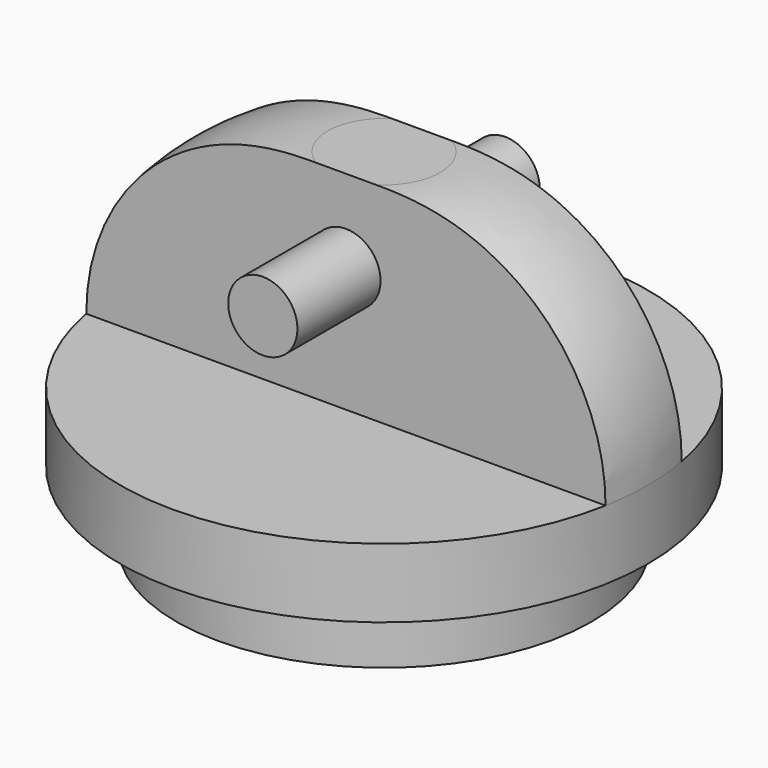
from build123d import *

# Parameters (mm, degrees)
F0_R        = 30
F1_DEPTH    = 10
F2_R        = 38.1255
F2_R_2      = 30
F3_DEPTH    = 10
F5_DEPTH    = 10
F7_DEPTH    = 20
F8_T2_ANGLE = 246.2138015041
F8_T4_ANGLE = 246.2138015041
F10_R       = 5
F11_DEPTH   = 15
F9_R        = 5
F12_DEPTH   = 15


# Not quite as in the source:
# - a fillet or chamfer that OpenCascade refuses, or shapes differently, is made with other operations: its cross-section is extruded or revolved along the edge and cut away or added


with BuildPart() as f1:
    # F0 (on Top) → F1 (new body)
    with BuildSketch(Plane.XY):
        Circle(F0_R)
    extrude(amount=F1_DEPTH)

    # F2 (on face) → F3 (join)
    with BuildSketch(Plane.XY.offset(10)):
        Circle(F2_R)
        Circle(F2_R_2, mode=Mode.SUBTRACT)
        Circle(F2_R_2)
    extrude(amount=F3_DEPTH)

    # F4 (on face) → F5 (join)
    with BuildSketch(Plane.XY.offset(20)):
        with BuildLine():
            Line((37.5, 6.8777721865), (-37.5, 6.8777721865))
            ThreePointArc((-37.5, 6.8777721865), (-38.1255, 0), (-37.5, -6.8777721865))
            Line((-37.5, -6.8777721865), (37.5, -6.8777721865))
            ThreePointArc((37.5, -6.8777721865), (37.9688029851, -3.4530783549), (38.1255, 0))
            ThreePointArc((38.1255, 0), (37.9688029851, 3.4530783549), (37.5, 6.8777721865))
        make_face()
    extrude(amount=F5_DEPTH)

    # F6 (on face) → F7 (join)
    with BuildSketch(Plane.XY.offset(30)):
        with BuildLine():
            Line((37.5, 6.8777721865), (-37.5, 6.8777721865))
            ThreePointArc((-37.5, 6.8777721865), (-38.1255, 0), (-37.5, -6.8777721865))
            Line((-37.5, -6.8777721865), (37.5, -6.8777721865))
            ThreePointArc((37.5, -6.8777721865), (38.1255, 0), (37.5, 6.8777721865))
        make_face()
    extrude(amount=F7_DEPTH)

    # F8: fillet of radius 30 on 2 edges, made by hand

    # F8_s1 → F8_t2 (revolve, cut)
    with BuildSketch(Plane(origin=(0, 0, 0), x_dir=(0, 0, 1), z_dir=(-0.8376529376, 0.5462028526, 0))):
        with BuildLine():
            ThreePointArc((20, -38.1255), (41.2132034356, -29.3387034356), (50, -8.1255))
            Line((50, -8.1255), (50, -38.1255))
            Line((50, -38.1255), (20, -38.1255))
        make_face()
    revolve(axis=Axis((0, 0, 50), (0, 0, 1)), revolution_arc=F8_T2_ANGLE, mode=Mode.SUBTRACT)

    # F8_s3 → F8_t4 (revolve, cut)
    with BuildSketch(Plane(origin=(0, 0, 0), x_dir=(0, 0, 1), z_dir=(0.8376529376, -0.5462028526, 0))):
        with BuildLine():
            ThreePointArc((20, -38.1255), (41.2132034356, -29.3387034356), (50, -8.1255))
            Line((50, -8.1255), (50, -38.1255))
            Line((50, -38.1255), (20, -38.1255))
        make_face()
    revolve(axis=Axis((0, 0, 50), (0, 0, 1)), revolution_arc=F8_T4_ANGLE, mode=Mode.SUBTRACT)

    # F10 (on face) → F11 (join)
    with BuildSketch(Plane(origin=(0, 6.8777721865, 0), x_dir=(-1, 0, 0), z_dir=(0, 1, 0))):
        with Locations((0, 38)):
            Circle(F10_R)
    extrude(amount=F11_DEPTH)

    # F9 (on face) → F12 (join)
    with BuildSketch(Plane.XZ.offset(6.8777721865)):
        with Locations((0, 38)):
            Circle(F9_R)
    extrude(amount=F12_DEPTH)


solid = f1.part
